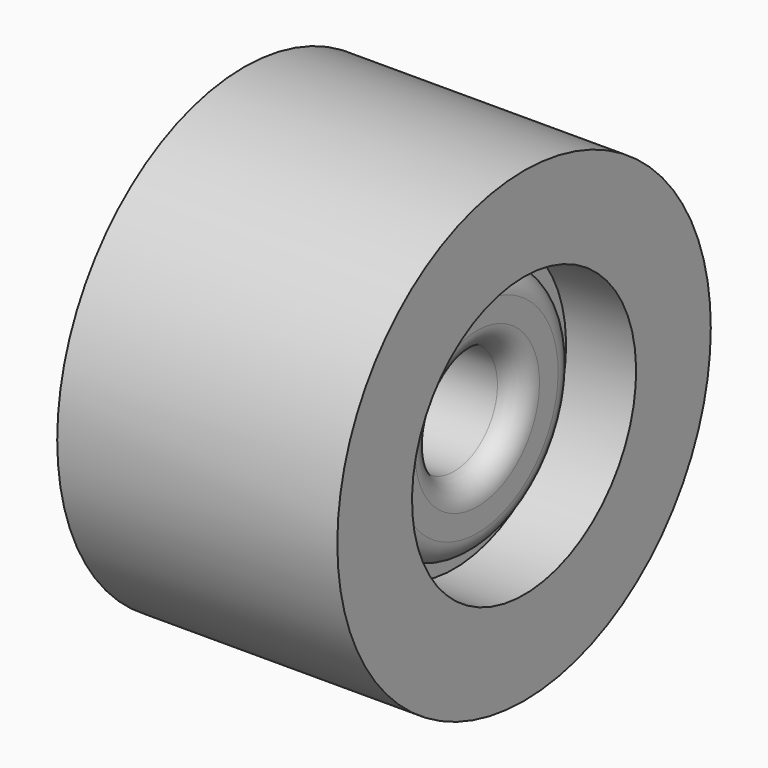
from build123d import *

# Parameters (mm, degrees)
F2_R = 4.99999


# Not quite as in the source:
# - a fillet or chamfer is up to 0.001 mm smaller than in the source, because OpenCascade refuses the exact size


with BuildPart() as f1:
    # F0 (on Front) → F1 (revolve)
    with BuildSketch(Plane.XZ):
        Polygon((-20, 11.6256596521), (0, 11.6256596521), (20, 11.6256596521), (20, 26.6256596521), (15, 26.6256596521), (15, 30), (30, 30), (30, 50), (0, 50), (-30, 50), (-30, 30), (-15, 30), (-15, 26.6256596521), (-20, 26.6256596521), align=None)
    revolve(axis=Axis((30.7941585779, 0, 0), (1, 0, 0)))

    # F2 (radius 5 in the source; OpenCascade refuses exactly that, so slightly less here)
    f2_edges = [f1.edges().sort_by_distance(p)[0] for p in [
        (20, 0, -11.62566),
        (20, 0, -26.62566),
    ]]
    fillet(f2_edges, radius=F2_R)


solid = f1.part
